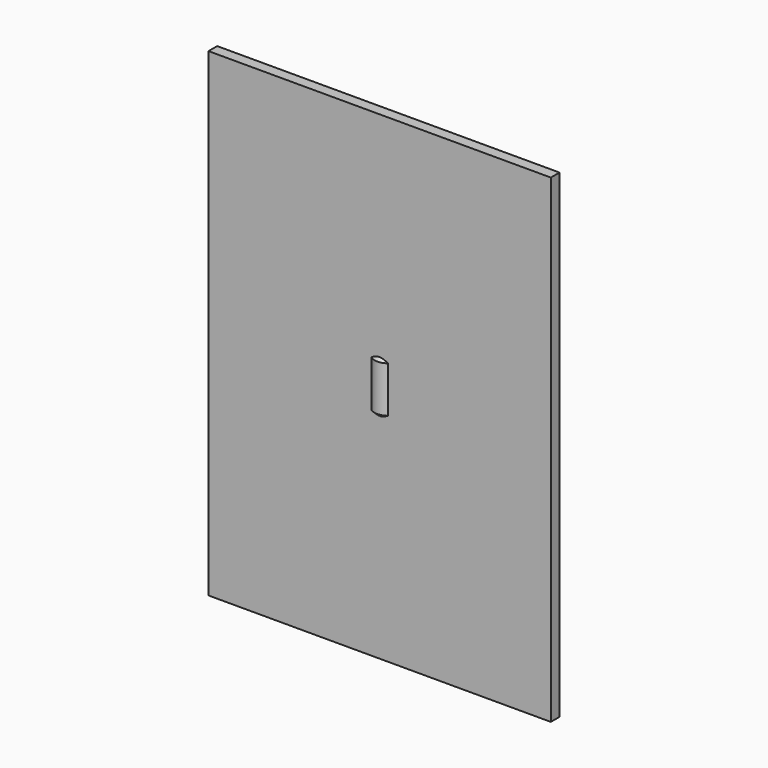
from build123d import *

# Parameters (mm, degrees)
F0_R     = 2
F1_DEPTH = 4
F2_SIZE  = 0.63
F3_W     = 50
F3_H     = 70
F4_DEPTH = 1.5875


# Not quite as in the source:
# - a length typed as a fraction of an inch, garbled in the dataset ("3 / 203.2 mm" for 3/8 in), is restored


with BuildPart() as f1:
    # F0 (on Top) → F1 (new body, symmetric)
    with BuildSketch(Plane.XY):
        Circle(F0_R)
    extrude(amount=F1_DEPTH, both=True)

    # F2
    f2_edges = [f1.edges().sort_by_distance(p)[0] for p in [
        (-2, 0, 4),
        (-2, 0, -4),
    ]]
    chamfer(f2_edges, length=F2_SIZE)


with BuildPart() as f4:
    # F3 (on Front) → F4 (new body)
    with BuildSketch(Plane.XZ):
        Rectangle(F3_W, F3_H)
    extrude(amount=F4_DEPTH)


solid = Compound([f1.part, f4.part])
